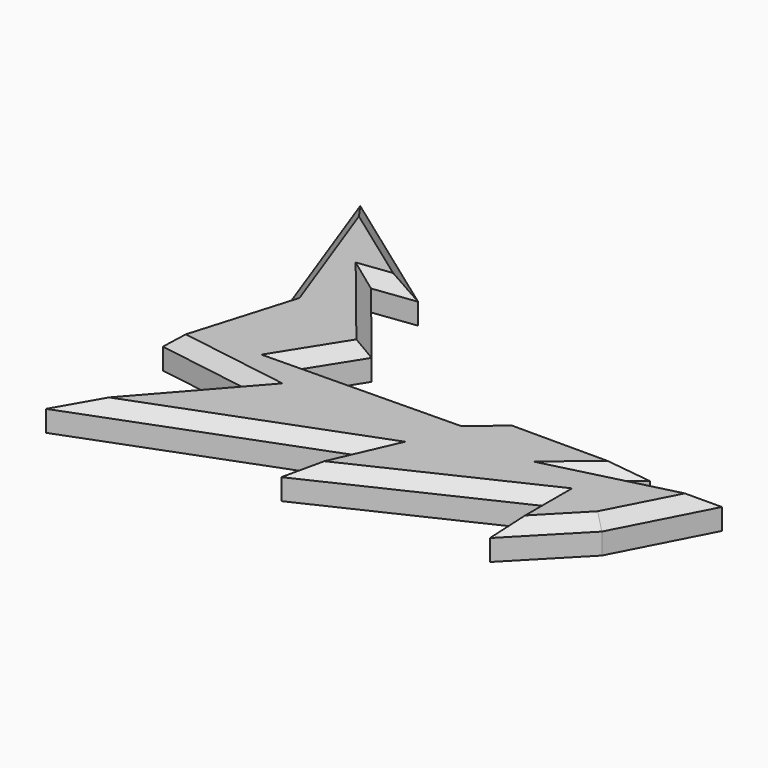
from build123d import *

# Parameters (mm, degrees)
F1_DEPTH = 12.7
F2_SIZE  = 4.572


# Not quite as in the source:
# - a feature names something its author has since deleted; it is built from what else it names


with BuildPart() as f1:
    # F0 (on Top) → F1 (new body)
    with BuildSketch(Plane.XY):
        Polygon((-138.7197226286, 19.6580234915), (-180.3987026215, -27.6248455048), (-85.8329609036, 8.0999890342), (-97.3909944296, -18.1682743132), (-23.6561261117, 16.663254671), (-23.6561261117, -9.9510056898), (0, 14.3561139703), (18.1893575937, 49.4287200272), (-20.6876713783, 39.6219007671), (-9.3052154407, 49.093272537), (-60.4820251465, 49.093272537), (-72.0571577549, 39.281655103), (-138.0494087934, 38.2558703423), (-124.7141808271, 59.4554506242), (-153.0797034502, 94.610132277), (-136.6182565689, 96.7115908861), (-189.1547888517, 134.5378756523), (-165.3382331133, 69.3925991654), (-178.2972365618, 25.9624067694), align=None)
    extrude(amount=F1_DEPTH)

    # F2
    f2_edges = [f1.edges().sort_by_distance(p)[0] for p in [
        (-162.886523, 115.624733, 12.7),
        (-177.246511, 101.965237, 12.7),
        (-171.817735, 47.677503, 12.7),
        (-158.50848, 22.810215, 12.7),
        (-159.559213, -3.983411, 12.7),
        (-133.115832, -9.762428, 12.7),
        (-91.611978, -5.034143, 12.7),
        (-60.52356, -0.75251, 12.7),
        (-23.656126, 3.356124, 12.7),
        (-11.828063, 2.202554, 12.7),
        (9.094679, 31.892417, 12.7),
        (-1.249157, 44.52531, 12.7),
        (-14.996443, 44.357587, 12.7),
        (-34.89362, 49.093273, 12.7),
        (-66.269591, 44.187464, 12.7),
        (-105.053283, 38.768763, 12.7),
        (-131.381795, 48.85566, 12.7),
        (-138.896942, 77.032791, 12.7),
        (-144.84898, 95.660862, 12.7),
    ]]
    chamfer(f2_edges, length=F2_SIZE)


solid = f1.part
